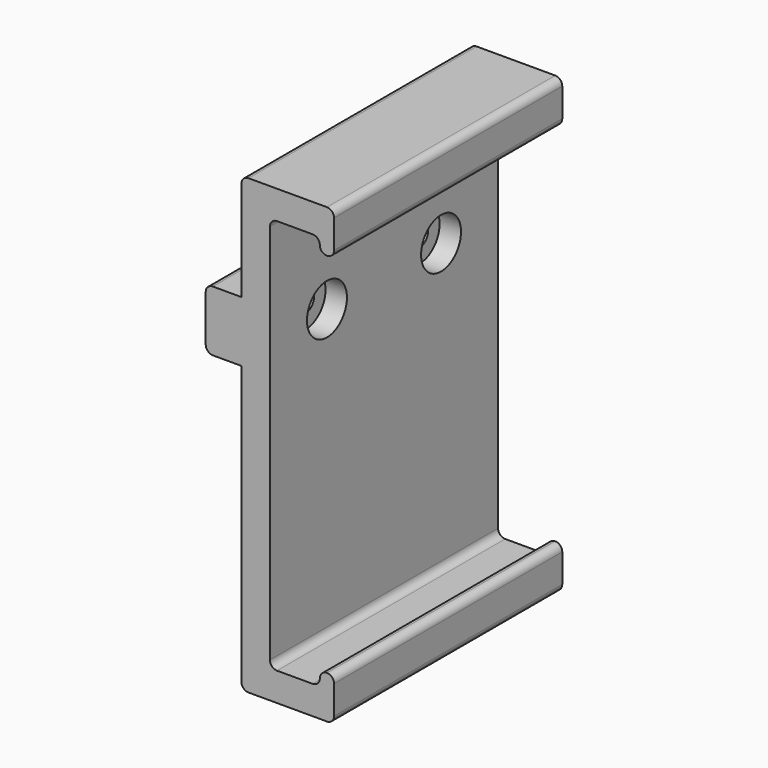
from build123d import *

# Parameters (mm, degrees)
F1_DEPTH = 40
F2_R     = 1.5
F3_DEPTH = 25
F5_R     = 1
F4_R     = 3.5
F4_R_2   = 1.5
F6_DEPTH = 3
F7_R     = 0.99999


# Not quite as in the source:
# - a fillet or chamfer is up to 0.001 mm smaller than in the source, because OpenCascade refuses the exact size


with BuildPart() as f1:
    # F0 (on Front) → F1 (new body)
    with BuildSketch(Plane.XZ):
        Polygon((13, 15), (0, 15), (0, 0), (-5, 0), (-5, -8.5), (0, -8.5), (0, -48.5), (13, -48.5), (13, -42.5), (11, -42.5), (11, -44.5), (4, -44.5), (4, 11), (11, 11), (11, 9), (13, 9), align=None)
    extrude(amount=F1_DEPTH)

    # F2 (on face) → F3 (cut)
    with BuildSketch(Plane(origin=(-5, 0, 0), x_dir=(0, -1, 0), z_dir=(-1, 0, 0))):
        with Locations((10, -4.25)):
            Circle(F2_R)
        with Locations((30, -4.25)):
            Circle(F2_R)
    extrude(amount=-F3_DEPTH, mode=Mode.SUBTRACT)

    # F5
    f5_edges = [f1.edges().sort_by_distance(p)[0] for p in [
        (-5, -20, 0),
        (-5, -20, -8.5),
    ]]
    fillet(f5_edges, radius=F5_R)

    # F4 (on face) → F6 (cut)
    with BuildSketch(Plane.YZ.offset(4)):
        with Locations((-10, -4.25)):
            Circle(F4_R)
        with Locations((-10, -4.25)):
            Circle(F4_R_2, mode=Mode.SUBTRACT)
        with Locations((-30, -4.25)):
            Circle(F4_R)
        with Locations((-30, -4.25)):
            Circle(F4_R_2, mode=Mode.SUBTRACT)
    extrude(amount=-F6_DEPTH, mode=Mode.SUBTRACT)

    # F7 (radius 1 in the source; OpenCascade refuses exactly that, so slightly less here)
    f7_edges = [f1.edges().sort_by_distance(p)[0] for p in [
        (13, -20, 9),
        (11, -20, 9),
        (13, -20, 15),
        (0, -20, 15),
        (4, -20, 11),
        (0, -20, -48.5),
        (13, -20, -48.5),
        (13, -20, -42.5),
        (4, -20, -44.5),
        (11, -20, -42.5),
        (11, -20, -44.5),
        (11, -20, 11),
    ]]
    fillet(f7_edges, radius=F7_R)


solid = f1.part
